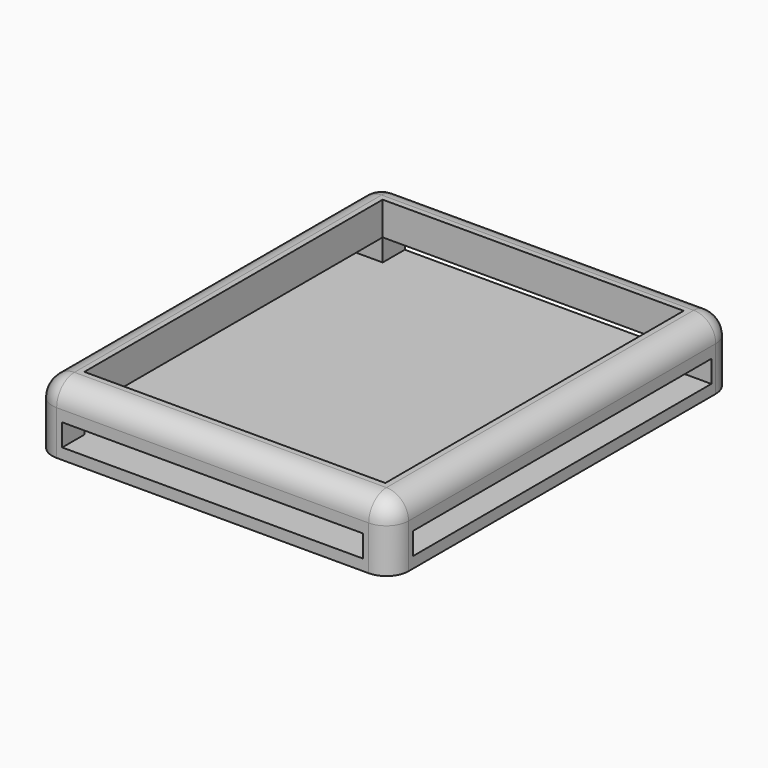
from build123d import *

# Parameters (mm, degrees)
F0_W         = 27.2
F0_H         = 2.5
F0_W_2       = 2.5
F0_H_2       = 33.7
F1_DEPTH     = 3
F2_R         = 2
F3_DEPTH     = 2
F4_W         = 2.5
F4_H         = 2.5
F5_DEPTH     = 1
F6_T1_DEPTH  = 9
F6_S5_W      = 2
F6_S5_H      = 2
F6_T6_DEPTH  = 2
F6_S11_W     = 2
F6_S11_H     = 2
F6_T12_DEPTH = 2
F6_S17_W     = 2
F6_S17_H     = 2
F6_T18_DEPTH = 2
F6_S23_W     = 2
F6_S23_H     = 2
F6_T24_DEPTH = 2


# Not quite as in the source:
# - a fillet or chamfer that OpenCascade refuses, or shapes differently, is made with other operations: its cross-section is extruded or revolved along the edge and cut away or added


with BuildPart() as f1:
    # F0 (on Top) → F1 (new body)
    with BuildSketch(Plane.XY):
        with Locations((0.1669520199, 18.5940534235)):
            Rectangle(F0_W, F0_H)
        with Locations((-14.6830479801, 0.4940534235)):
            Rectangle(F0_W_2, F0_H_2)
        with Locations((-14.6830479801, 18.5940534235)):
            Rectangle(F0_W_2, F0_H)
        with Locations((-14.6830479801, -17.6059465765)):
            Rectangle(F0_W_2, F0_H)
        with Locations((0.1669520199, -17.6059465765)):
            Rectangle(F0_W, F0_H)
        with Locations((15.0169520199, -17.6059465765)):
            Rectangle(F0_W_2, F0_H)
        with Locations((15.0169520199, 0.4940534235)):
            Rectangle(F0_W_2, F0_H_2)
        with Locations((15.0169520199, 18.5940534235)):
            Rectangle(F0_W_2, F0_H)
    extrude(amount=F1_DEPTH)

    # F2
    f2_edges = [f1.edges().sort_by_distance(p)[0] for p in [
        (16.266952, 0.494053, 3),
        (0.166952, 19.844053, 3),
        (-15.933048, 0.494053, 3),
        (0.166952, -18.855947, 3),
    ]]
    fillet(f2_edges, radius=F2_R)

    # F0 (on Top) → F3 (join)
    with BuildSketch(Plane.XY):
        with Locations((-14.6830479801, -17.6059465765)):
            Rectangle(F0_W_2, F0_H)
        with Locations((15.0169520199, -17.6059465765)):
            Rectangle(F0_W_2, F0_H)
        with Locations((15.0169520199, 18.5940534235)):
            Rectangle(F0_W_2, F0_H)
        with Locations((-14.6830479801, 18.5940534235)):
            Rectangle(F0_W_2, F0_H)
    extrude(amount=-F3_DEPTH)

    # F4 (on face) → F5 (join)
    with BuildSketch(Plane(origin=(0, 0, -2), x_dir=(1, 0, 0), z_dir=(0, 0, -1))):
        Polygon((-13.4330479801, -19.8440534235), (16.2669520199, -19.8440534235), (16.2669520199, 18.8559465765), (-15.9330479801, 18.8559465765), (-15.9330479801, -17.3440534235), (-13.4330479801, -17.3440534235), align=None)
        with Locations((-14.6830479801, -18.5940534235)):
            Rectangle(F4_W, F4_H)
    extrude(amount=F5_DEPTH)

    # F6: fillet of radius 2 on 4 edges, made by hand

    # F6_s2 → F6_t1 (cut)
    with BuildSketch(Plane.XY.offset(-8)):
        with BuildLine():
            ThreePointArc((16.2669520199, 17.8440534235), (15.6811655823, 19.2582669858), (14.2669520199, 19.8440534235))
            Line((14.2669520199, 19.8440534235), (16.2669520199, 19.8440534235))
            Line((16.2669520199, 19.8440534235), (16.2669520199, 17.8440534235))
        make_face()
        with BuildLine():
            ThreePointArc((16.2669520199, -16.8559465765), (15.6811655823, -18.2701601389), (14.2669520199, -18.8559465765))
            Line((14.2669520199, -18.8559465765), (16.2669520199, -18.8559465765))
            Line((16.2669520199, -18.8559465765), (16.2669520199, -16.8559465765))
        make_face()
        with BuildLine():
            ThreePointArc((-15.9330479801, -16.8559465765), (-15.3472615424, -18.2701601389), (-13.9330479801, -18.8559465765))
            Line((-13.9330479801, -18.8559465765), (-15.9330479801, -18.8559465765))
            Line((-15.9330479801, -18.8559465765), (-15.9330479801, -16.8559465765))
        make_face()
        with BuildLine():
            ThreePointArc((-15.9330479801, 17.8440534235), (-15.3472615424, 19.2582669858), (-13.9330479801, 19.8440534235))
            Line((-13.9330479801, 19.8440534235), (-15.9330479801, 19.8440534235))
            Line((-15.9330479801, 19.8440534235), (-15.9330479801, 17.8440534235))
        make_face()
    extrude(amount=F6_T1_DEPTH, mode=Mode.SUBTRACT)


with BuildPart() as f6_tool4:
    # F6_s5 → F6_t6 (new body)
    with BuildSketch(Plane.YZ.offset(-13.9330479801)):
        with Locations((18.8440534235, 2)):
            Rectangle(F6_S5_W, F6_S5_H)
    extrude(amount=-F6_T6_DEPTH)

    # F6_s7 → F6_t8 (revolve, cut)
    with BuildSketch(Plane(origin=(-13.9330479801, 17.8440534235, 1), x_dir=(0, -0.7071067812, -0.7071067812), z_dir=(0, 0.7071067812, -0.7071067812))):
        with BuildLine():
            ThreePointArc((0, -2), (2, 0), (0, 2))
            Line((0, 2), (0, -2))
        make_face()
    revolve(axis=Axis((-13.9330479801, 17.8440534235, 1), (-1, 0, 0)), mode=Mode.SUBTRACT)


with BuildPart() as f1_1:
    add(f1.part)

    # F6_t3: cut F6_tool4
    add(f6_tool4.part, mode=Mode.SUBTRACT)


with BuildPart() as f6_tool10:
    # F6_s11 → F6_t12 (new body)
    with BuildSketch(Plane.YZ.offset(-13.9330479801)):
        with Locations((-17.8559465765, 2)):
            Rectangle(F6_S11_W, F6_S11_H)
    extrude(amount=-F6_T12_DEPTH)

    # F6_s13 → F6_t14 (revolve, cut)
    with BuildSketch(Plane(origin=(-13.9330479801, -16.8559465765, 1), x_dir=(0, 0.7071067812, -0.7071067812), z_dir=(0, 0.7071067812, 0.7071067812))):
        with BuildLine():
            ThreePointArc((0, -2), (2, 0), (0, 2))
            Line((0, 2), (0, -2))
        make_face()
    revolve(axis=Axis((-13.9330479801, -16.8559465765, 1), (-1, 0, 0)), mode=Mode.SUBTRACT)


with BuildPart() as f1_2:
    add(f1_1.part)

    # F6_t9: cut F6_tool10
    add(f6_tool10.part, mode=Mode.SUBTRACT)


with BuildPart() as f6_tool16:
    # F6_s17 → F6_t18 (new body)
    with BuildSketch(Plane.YZ.offset(14.2669520199)):
        with Locations((-17.8559465765, 2)):
            Rectangle(F6_S17_W, F6_S17_H)
    extrude(amount=F6_T18_DEPTH)

    # F6_s19 → F6_t20 (revolve, cut)
    with BuildSketch(Plane(origin=(14.2669520199, -16.8559465765, 1), x_dir=(0, 0.7071067812, -0.7071067812), z_dir=(0, -0.7071067812, -0.7071067812))):
        with BuildLine():
            ThreePointArc((0, -2), (2, 0), (0, 2))
            Line((0, 2), (0, -2))
        make_face()
    revolve(axis=Axis((14.2669520199, -16.8559465765, 1), (1, 0, 0)), mode=Mode.SUBTRACT)


with BuildPart() as f1_3:
    add(f1_2.part)

    # F6_t15: cut F6_tool16
    add(f6_tool16.part, mode=Mode.SUBTRACT)


with BuildPart() as f6_tool22:
    # F6_s23 → F6_t24 (new body)
    with BuildSketch(Plane.YZ.offset(14.2669520199)):
        with Locations((18.8440534235, 2)):
            Rectangle(F6_S23_W, F6_S23_H)
    extrude(amount=F6_T24_DEPTH)

    # F6_s25 → F6_t26 (revolve, cut)
    with BuildSketch(Plane(origin=(14.2669520199, 17.8440534235, 1), x_dir=(0, -0.7071067812, -0.7071067812), z_dir=(0, -0.7071067812, 0.7071067812))):
        with BuildLine():
            ThreePointArc((0, -2), (2, 0), (0, 2))
            Line((0, 2), (0, -2))
        make_face()
    revolve(axis=Axis((14.2669520199, 17.8440534235, 1), (1, 0, 0)), mode=Mode.SUBTRACT)


with BuildPart() as f1_4:
    add(f1_3.part)

    # F6_t21: cut F6_tool22
    add(f6_tool22.part, mode=Mode.SUBTRACT)


solid = f1_4.part
